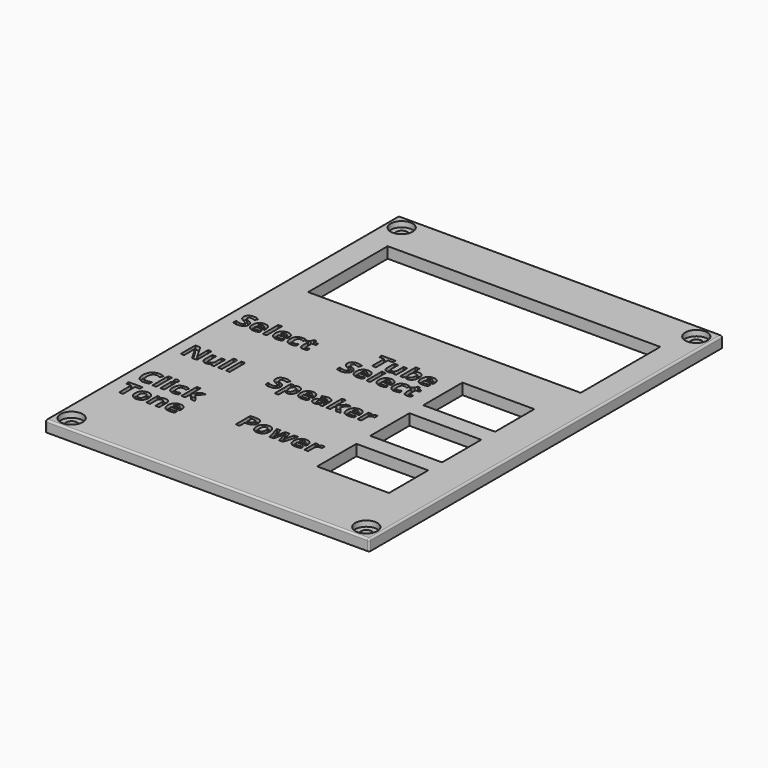
from build123d import *

# Parameters (mm, degrees)
F0_W           = 88
F0_H           = 120
F0_W_2         = 19.5
F0_H_2         = 13.3
F0_W_3         = 74
F0_H_3         = 27
F1_DEPTH       = 3
F3_D           = 3
F3_CBORE_D     = 6
F3_CBORE_DEPTH = 1.5
F4_TEXT_SIZE   = 6.9444444444
F5_DEPTH       = 1
F6_R           = 0.5


# Not quite as in the source:
# - Text() gives the source's letters only with a copy of the font that has no kerning and outlines rounded to 1/6400 em; it was checked with that copy


with BuildPart() as f1:
    # F0 (on Top) → F1 (new body)
    with BuildSketch(Plane.XY):
        with Locations((44, 60)):
            Rectangle(F0_W, F0_H)
        with Locations((68.25, 25.85)):
            Rectangle(F0_W_2, F0_H_2, mode=Mode.SUBTRACT)
        with Locations((68.25, 43.85)):
            Rectangle(F0_W_2, F0_H_2, mode=Mode.SUBTRACT)
        with Locations((68.25, 61.85)):
            Rectangle(F0_W_2, F0_H_2, mode=Mode.SUBTRACT)
        with Locations((44, 94)):
            Rectangle(F0_W_3, F0_H_3, mode=Mode.SUBTRACT)
    extrude(amount=F1_DEPTH)

    # F3 (through all)
    with Locations(Plane.XY.offset(3)):
        with Locations((4, 116), (84, 116), (84, 4), (4, 4)):
            CounterBoreHole(F3_D / 2, F3_CBORE_D / 2, F3_CBORE_DEPTH)

    # F4 (on face) → F5 (cut)
    with BuildSketch(Plane.XY.offset(3)):
        with Locations((37.2658420139, 62.5)):
            Text('Tube', F4_TEXT_SIZE, font='Open Sans', font_style=FontStyle.BOLD, text_align=(TextAlign.LEFT, TextAlign.BOTTOM))
        with Locations((33.5386284722, 56.5)):
            Text('Select', F4_TEXT_SIZE, font='Open Sans', font_style=FontStyle.BOLD, text_align=(TextAlign.LEFT, TextAlign.BOTTOM))
        with Locations((32.3342013889, 23.5)):
            Text('Power', F4_TEXT_SIZE, font='Open Sans', font_style=FontStyle.BOLD, text_align=(TextAlign.LEFT, TextAlign.BOTTOM))
        with Locations((26.1156684028, 41.5)):
            Text('Speaker', F4_TEXT_SIZE, font='Open Sans', font_style=FontStyle.BOLD, text_align=(TextAlign.LEFT, TextAlign.BOTTOM))
        with Locations((3, 59.5)):
            Text('Select', F4_TEXT_SIZE, font='Open Sans', font_style=FontStyle.BOLD, text_align=(TextAlign.LEFT, TextAlign.BOTTOM))
        with Locations((3, 41.5)):
            Text('Null', F4_TEXT_SIZE, font='Open Sans', font_style=FontStyle.BOLD, text_align=(TextAlign.LEFT, TextAlign.BOTTOM))
        with Locations((3, 26.5)):
            Text('Click', F4_TEXT_SIZE, font='Open Sans', font_style=FontStyle.BOLD, text_align=(TextAlign.LEFT, TextAlign.BOTTOM))
        with Locations((3, 19.5)):
            Text('Tone', F4_TEXT_SIZE, font='Open Sans', font_style=FontStyle.BOLD, text_align=(TextAlign.LEFT, TextAlign.BOTTOM))
    extrude(amount=-F5_DEPTH, mode=Mode.SUBTRACT)

    # F6
    f6_edges = [f1.edges().sort_by_distance(p)[0] for p in [
        (0, 60, 3),
        (44, 120, 3),
        (88, 60, 3),
        (44, 0, 3),
        (0, 0, 1.5),
        (88, 0, 1.5),
        (0, 120, 1.5),
        (88, 120, 1.5),
    ]]
    fillet(f6_edges, radius=F6_R)


solid = f1.part
